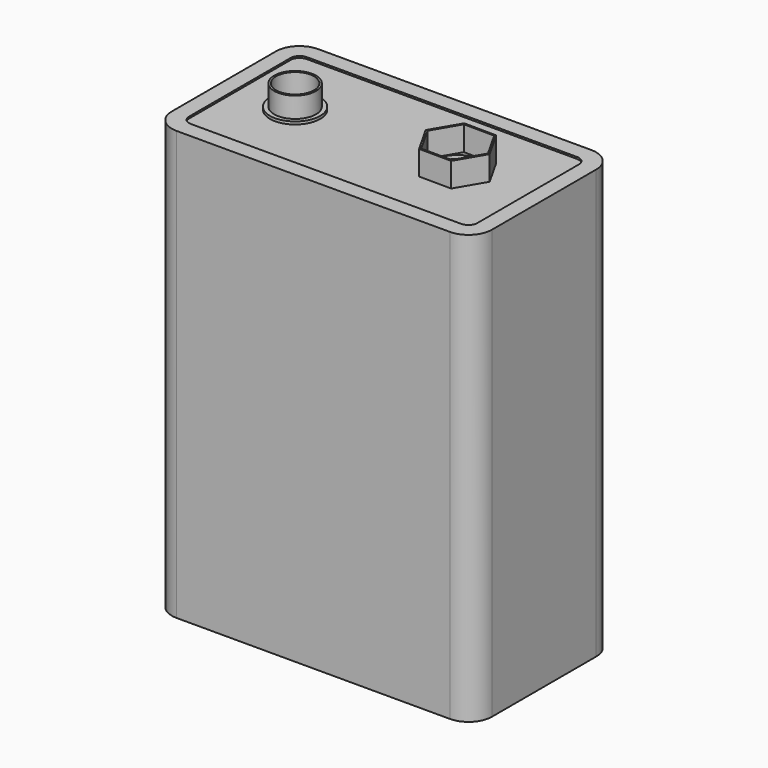
from build123d import *

# Parameters (mm, degrees)
F0_W      = 45.1385900378
F0_H      = 24.9742213637
F1_DEPTH  = 30.226
F2_R      = 3.302
F3_W      = 40.6467653811
F3_H      = 20.4270016402
F4_DEPTH  = 0.254
F5_R      = 1.27
F6_R      = 2.9461453385
F7_DEPTH  = 3.2766
F6_R_2    = 3.5430744691
F8_DEPTH  = 0.381
F9_DEPTH  = 3.429
F11_DEPTH = 3.4544
F12_R     = 3.565401554
F13_DEPTH = 0.508
F14_R     = 0.4846078425
F15_DEPTH = 0.0762
F14_R_2   = 1.0356451119
F16_DEPTH = 0.254
F18_R     = 2.6755593281
F18_R_2   = 0.8351552506
F19_DEPTH = 2.8702
F20_R     = 2.2091463804
F21_DEPTH = 4.3942


# Not quite as in the source:
# - a fillet or chamfer that OpenCascade refuses, or shapes differently, is made with other operations: its cross-section is extruded or revolved along the edge and cut away or added


with BuildPart() as f1:
    # F0 (on Top) → F1 (new body, symmetric)
    with BuildSketch(Plane.XY):
        Rectangle(F0_W, F0_H)
    extrude(amount=F1_DEPTH, both=True)

    # F2
    f2_edges = [f1.edges().sort_by_distance(p)[0] for p in [
        (-22.569295, -12.487111, 0),
        (-22.569295, 12.487111, 0),
        (22.569295, -12.487111, 0),
        (22.569295, 12.487111, 0),
    ]]
    fillet(f2_edges, radius=F2_R)

    # F3 (on face) → F4 (cut)
    with BuildSketch(Plane.XY.offset(30.226)):
        Rectangle(F3_W, F3_H)
    extrude(amount=-F4_DEPTH, mode=Mode.SUBTRACT)

    # F5
    f5_edges = [f1.edges().sort_by_distance(p)[0] for p in [
        (-20.323383, 10.213501, 30.099),
        (-20.323383, -10.213501, 30.099),
        (20.323383, 10.213501, 30.099),
        (20.323383, -10.213501, 30.099),
    ]]
    fillet(f5_edges, radius=F5_R)

    # F6 (on face) → F7 (join)
    with BuildSketch(Plane.XY.offset(29.972)):
        with Locations((-12.5333582982, 0)):
            Circle(F6_R)
    extrude(amount=F7_DEPTH)

    # F6 (on face) → F8 (join)
    with BuildSketch(Plane.XY.offset(29.972)):
        with Locations((-12.5333582982, 0)):
            Circle(F6_R_2)
        with Locations((-12.5333582982, 0)):
            Circle(F6_R, mode=Mode.SUBTRACT)
    extrude(amount=F8_DEPTH)

    # F6 (on face) → F9 (join)
    with BuildSketch(Plane.XY.offset(29.972)):
        Polygon((12.6905003563, 3.9159879088), (8.1466763174, 3.9541461872), (5.8417182595, 0.0381582783), (8.0805842406, -3.9159879088), (12.6244082795, -3.9541461872), (14.9293663373, -0.0381582783), align=None)
    extrude(amount=F9_DEPTH)

    # F10 (on face) → F11 (cut)
    with BuildSketch(Plane.XY.offset(33.401)):
        Polygon((12.5692944355, 3.700253209), (8.275793058, 3.7363093193), (6.0978168617, 0.0360561103), (8.213342043, -3.700253209), (12.5068434206, -3.7363093193), (14.6848196168, -0.0360561103), align=None)
    extrude(amount=-F11_DEPTH, mode=Mode.SUBTRACT)

    # F12 (on face) → F13 (cut)
    with BuildSketch(Plane.XY.offset(29.972)):
        with Locations((10.3914178908, 0)):
            Circle(F12_R)
    extrude(amount=-F13_DEPTH, mode=Mode.SUBTRACT)

    # F18 (on face) → F19 (cut)
    with BuildSketch(Plane.XY.offset(33.2486)):
        with Locations((-12.5333582982, 0)):
            Circle(F18_R)
        with Locations((-12.5333582982, 0)):
            Circle(F18_R_2, mode=Mode.SUBTRACT)
    extrude(amount=-F19_DEPTH, mode=Mode.SUBTRACT)

    # F20 (on face) → F21 (cut)
    with BuildSketch(Plane.XY.offset(33.2486)):
        with Locations((-12.5184208155, 0)):
            Circle(F20_R)
    extrude(amount=-F21_DEPTH, mode=Mode.SUBTRACT)


with BuildPart() as f15:
    # F14 (on face) → F15 (new body)
    with BuildSketch(Plane.XY.offset(29.972)):
        with Locations((10.4190623388, 0)):
            Circle(F14_R)
    extrude(amount=F15_DEPTH)

    # F14 (on face) → F16 (join)
    with BuildSketch(Plane.XY.offset(29.972)):
        with Locations((10.4190623388, 0)):
            Circle(F14_R_2)
        with Locations((10.4190623388, 0)):
            Circle(F14_R, mode=Mode.SUBTRACT)
    extrude(amount=F16_DEPTH)

    # F17: fillet of radius 0.254 on 2 edges, made by hand

    # F17_s1 → F17_t2 (revolve, cut)
    with BuildSketch(Plane.XZ):
        with BuildLine():
            ThreePointArc((11.4547074506, 29.972), (11.380312573, 30.1516051224), (11.2007074506, 30.226))
            Line((11.2007074506, 30.226), (11.4547074506, 30.226))
            Line((11.4547074506, 30.226), (11.4547074506, 29.972))
        make_face()
    revolve(axis=Axis((10.4190623388, 0, 30.226), (0, 0, 1)), mode=Mode.SUBTRACT)

    # F17_s3 → F17_t4 (revolve, cut)
    with BuildSketch(Plane.XZ):
        with BuildLine():
            ThreePointArc((11.1459707384, 30.226), (10.9957023119, 30.1767813468), (10.9036701812, 30.0482))
            Line((10.9036701812, 30.0482), (10.9036701812, 30.226))
            Line((10.9036701812, 30.226), (11.1459707384, 30.226))
        make_face()
    revolve(axis=Axis((10.4190623388, 0, 30.226), (0, 0, 1)), mode=Mode.SUBTRACT)


solid = Compound([f1.part, f15.part])
